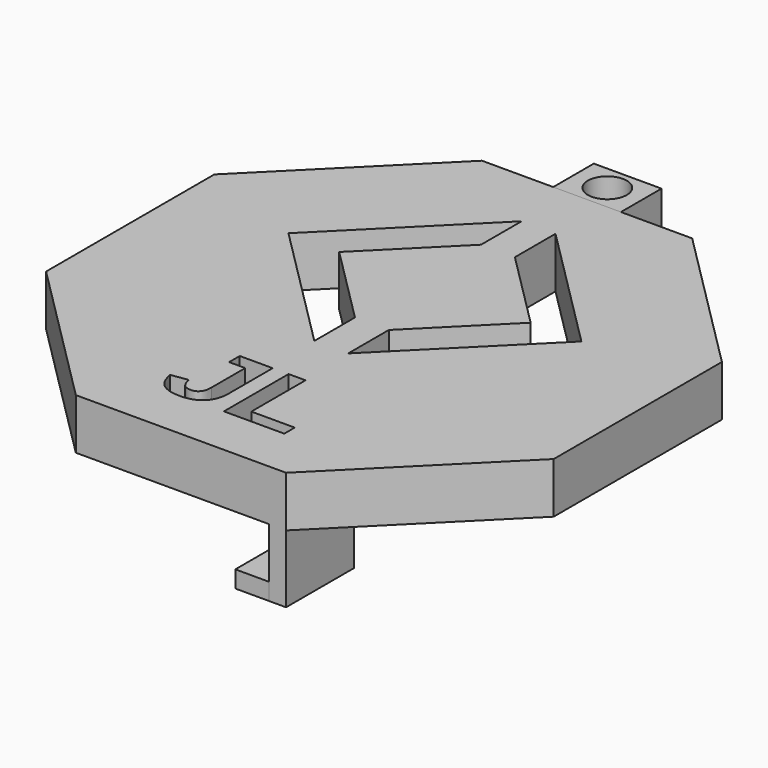
from build123d import *

# Parameters (mm, degrees)
F1_DEPTH     = 3
F2_TEXT_SIZE = 6.9444444444
F3_DEPTH     = 3.001
F4_W         = 1
F4_H         = 5
F5_DEPTH     = 4
F6_W         = 5
F6_H         = 1
F7_DEPTH     = 2
F8_W         = 4
F8_H         = 3
F9_DEPTH     = 3
F10_R        = 1.15
F11_DEPTH    = 3.0010001


# Not quite as in the source:
# - Text() gives the source's letters only with a copy of the font that has no kerning and outlines rounded to 1/6400 em; it was checked with that copy


with BuildPart() as f1:
    # F0 (on Top) → F1 (new body)
    with BuildSketch(Plane.XY):
        Polygon((15, -6.2132034356), (15, 6.2132034356), (6.2132034356, 15), (-6.2132034356, 15), (-15, 6.2132034356), (-15, -6.2132034356), (-6.2132034356, -15), (6.2132034356, -15), align=None)
    extrude(amount=F1_DEPTH)

    # F2 (on face) → F3 (cut, through all)
    with BuildSketch(Plane.XY.offset(3)):
        Polygon((1, 8.418436326), (5.6568542495, 3.7615820765), (1, -0.8952721729), (1, -3.8952721729), (8.6568542495, 3.7615820765), (1, 11.418436326), align=None)
        Polygon((-1, -0.8952721729), (-5.6568542495, 3.7615820765), (-1, 8.418436326), (-1, 11.418436326), (-8.6568542495, 3.7615820765), (-1, -3.8952721729), align=None)
        with Locations((-4.1861979167, -12)):
            Text('JL', F2_TEXT_SIZE, font='Arimo', font_style=FontStyle.BOLD, text_align=(TextAlign.LEFT, TextAlign.BOTTOM))
    extrude(amount=-F3_DEPTH, mode=Mode.SUBTRACT)

    # F4 (on face) → F5 (join)
    with BuildSketch(Plane(origin=(0, 0, 0), x_dir=(1, 0, 0), z_dir=(0, 0, -1))):
        with Locations((5.7132034356, 12.5)):
            Rectangle(F4_W, F4_H)
    extrude(amount=F5_DEPTH)


with BuildPart() as f7:
    # F6 (on face) → F7 (new body)
    with BuildSketch(Plane(origin=(5.2132034356, 0, 0), x_dir=(0, -1, 0), z_dir=(-1, 0, 0))):
        with Locations((12.5, -3.5)):
            Rectangle(F6_W, F6_H)
    extrude(amount=F7_DEPTH)


with BuildPart() as f9:
    # F8 (on face) → F9 (new body)
    with BuildSketch(Plane(origin=(0, 15, 0), x_dir=(-1, 0, 0), z_dir=(0, 1, 0))):
        with Locations((0, 1.5)):
            Rectangle(F8_W, F8_H)
    extrude(amount=F9_DEPTH)

    # F10 (on face) → F11 (cut, through all)
    with BuildSketch(Plane(origin=(0, 0, 0), x_dir=(1, 0, 0), z_dir=(0, 0, -1))):
        with Locations((0, -16.5)):
            Circle(F10_R)
    extrude(amount=-F11_DEPTH, mode=Mode.SUBTRACT)


solid = Compound([f1.part, f7.part, f9.part])
